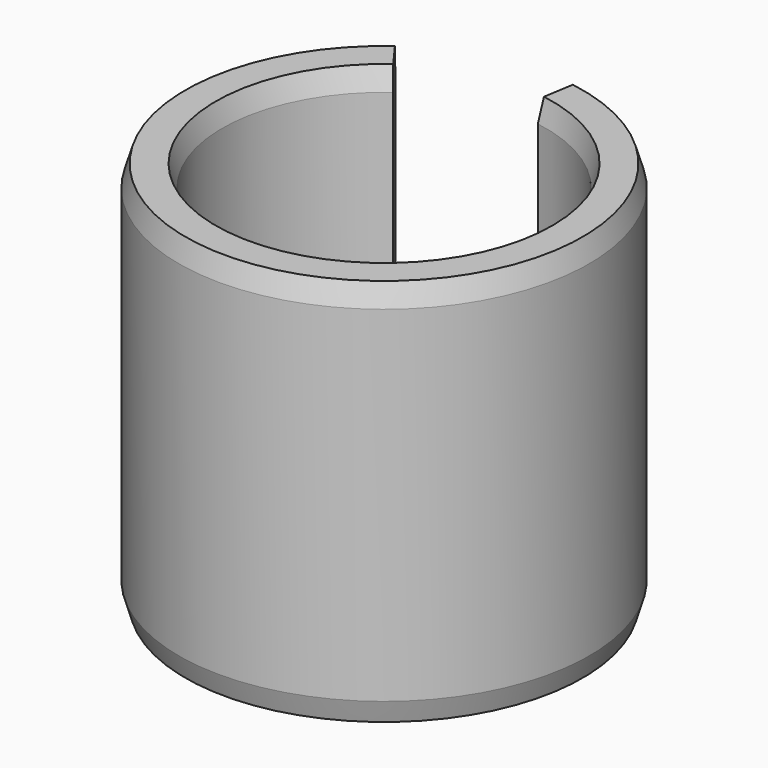
from build123d import *

# Parameters (mm, degrees)
F1_DEPTH   = 18
F2_SIZE2   = 1
F2_SIZE    = 0.3
F2_2_SIZE2 = 1
F2_2_SIZE  = 0.3


# Not quite as in the source:
# - a feature names something its author has since deleted; it is built from what else it names


with BuildPart() as f1:
    # F0 (on Top) → F1 (new body)
    with BuildSketch(Plane.XY):
        with BuildLine():
            ThreePointArc((1.2044566856, 7.40527886), (1.7499452086, -7.2956536834), (-4.4326164701, 6.0531629856))
            Line((-4.4326164701, 6.0531629856), (-5.6190034408, 7.6732881976))
            ThreePointArc((-5.6190034408, 7.6732881976), (2.2183169274, -9.2483307381), (1.5268287492, 9.3872970232))
            Line((1.5268287492, 9.3872970232), (1.2044566856, 7.40527886))
        make_face()
    extrude(amount=F1_DEPTH)

    # F2
    f2_edges = [f1.edges().sort_by_distance(p)[0] for p in [
        (2.218317, -9.248331, 18),
        (1.749945, -7.295654, 18),
    ]]
    f2_side = f1.faces().sort_by_distance((1.630296, 8.353243, 18))[0]
    chamfer(f2_edges, length=F2_SIZE, length2=F2_SIZE2, reference=f2_side)

    # F2#2
    f2_2_edges = [f1.edges().sort_by_distance(p)[0] for p in [
        (2.218317, -9.248331, 0),
        (1.749945, -7.295654, 0),
    ]]
    f2_2_side = f1.faces().sort_by_distance((1.630296, 8.353243, 0))[0]
    chamfer(f2_2_edges, length=F2_2_SIZE, length2=F2_2_SIZE2, reference=f2_2_side)


solid = f1.part
